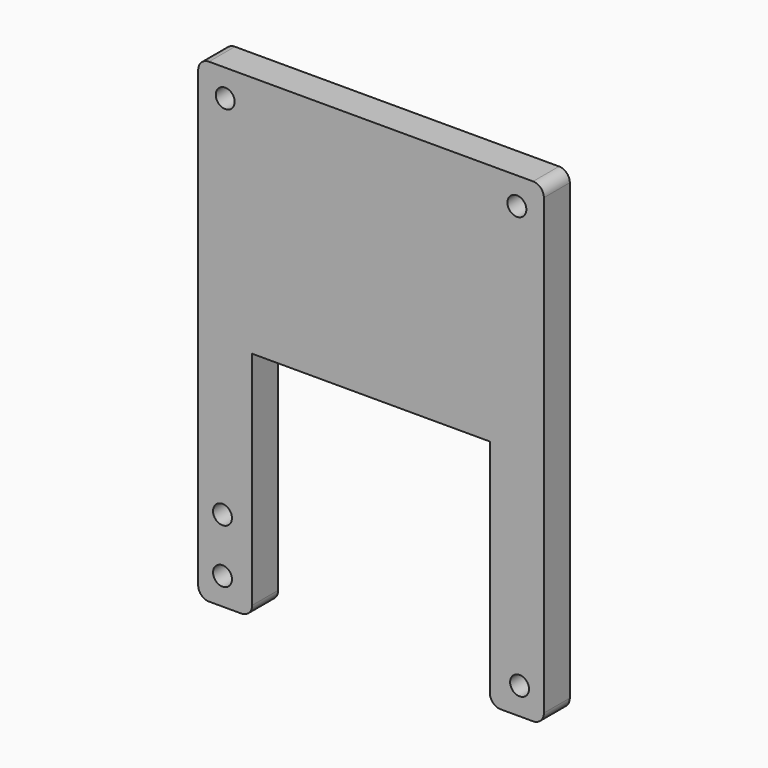
from build123d import *

# Parameters (mm, degrees)
F0_W     = 64
F0_H     = 88
F1_DEPTH = 6
F2_R     = 1.75
F3_DEPTH = 25
F4_R     = 2


# Not quite as in the source:
# - a feature names something its author has since deleted; it is built from what else it names


with BuildPart() as f1:
    # F0 (on Front) → F1 (new body)
    with BuildSketch(Plane.XZ):
        Rectangle(F0_W, F0_H)
    extrude(amount=F1_DEPTH)

    # F2 (on face) → F3 (cut)
    with BuildSketch(Plane.XZ.offset(6)):
        Polygon((22, -1), (0, -1), (-22, -1), (-22, -44), (22, -44), align=None)
        with Locations((27.5, -39)):
            Circle(F2_R)
        with Locations((-27.5, -29)):
            Circle(F2_R)
        with Locations((-27.5, -39)):
            Circle(F2_R)
        with Locations((-27, 39)):
            Circle(F2_R)
        with Locations((27, 39)):
            Circle(F2_R)
    extrude(amount=-F3_DEPTH, mode=Mode.SUBTRACT)

    # F4
    f4_edges = [f1.edges().sort_by_distance(p)[0] for p in [
        (-32, -3, 44),
        (32, -3, 44),
        (-32, -3, -44),
        (32, -3, -44),
        (-22, -3, -44),
        (22, -3, -44),
    ]]
    fillet(f4_edges, radius=F4_R)


solid = f1.part
